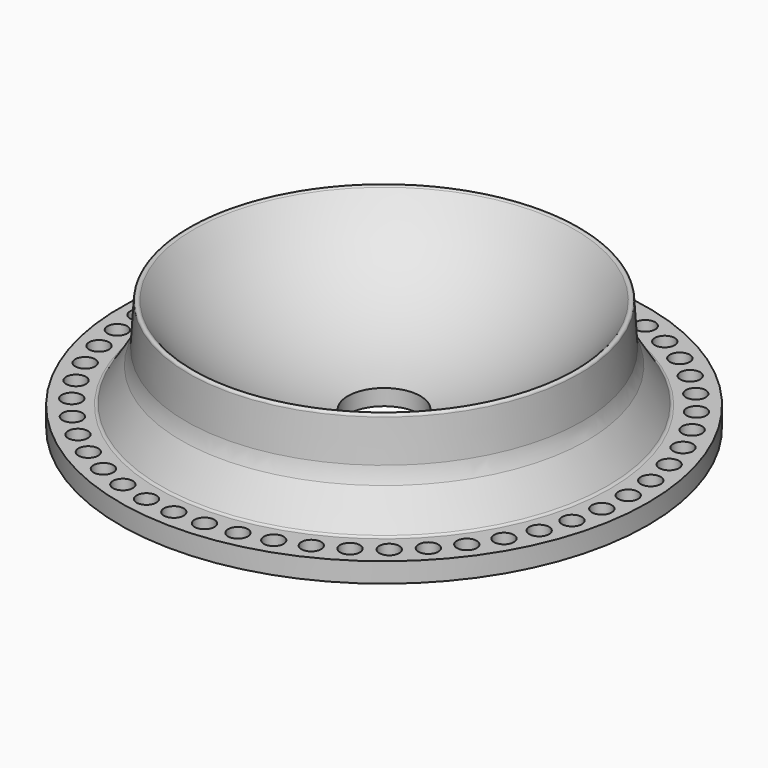
from build123d import *

# Parameters (mm, degrees)
F2_R            = 0.4
F3_R            = 5
F4_R            = 0.5
F5_R            = 5.5
F6_DEPTH        = 2.4321027845
F7_R            = 1.5
F8_DEPTH        = 3
F8_COPIES_COUNT = 50


# Not quite as in the source:
# - a pattern or mirror of a feature is missing from the dataset's text; its kind, count and spacing are read off the source's solid


with BuildPart() as f1:
    # F0 (on Front) → F1 (revolve)
    with BuildSketch(Plane.XZ):
        with BuildLine():
            Line((0, 2), (0, 0))
            Line((0, 0), (40, 0))
            Line((40, 0), (40, 3))
            Line((40, 3), (34, 3))
            Line((34, 3), (30.0883166492, 9.3437703326))
            Line((30.0883166492, 9.3437703326), (29.5567251231, 18))
            ThreePointArc((29.5567251231, 18), (16.8047612301, 6.2566432227), (0, 2))
        make_face()
    revolve(axis=Axis((0, 0, 1), (0, 0, -1)))

    # F2
    f2_edges = [f1.edges().sort_by_distance(p)[0] for p in [
        (-29.556725, 0, 18),
    ]]
    fillet(f2_edges, radius=F2_R)

    # F3
    f3_edges = [f1.edges().sort_by_distance(p)[0] for p in [
        (-30.088317, 0, 9.34377),
    ]]
    fillet(f3_edges, radius=F3_R)

    # F4
    f4_edges = [f1.edges().sort_by_distance(p)[0] for p in [
        (-34, 0, 3),
    ]]
    fillet(f4_edges, radius=F4_R)

    # F5 (on face) → F6 (cut, through all)
    with BuildSketch(Plane(origin=(0, 0, 0), x_dir=(1, 0, 0), z_dir=(0, 0, -1))):
        Circle(F5_R)
    extrude(amount=-F6_DEPTH, mode=Mode.SUBTRACT)

    # F7 (on face) → F8 (cut, through all)
    with BuildSketch(Plane.XY.offset(3)):
        with Locations((37, 0)):
            Circle(F7_R)
    f8 = extrude(amount=-F8_DEPTH, mode=Mode.SUBTRACT)

    # F8_copies: F8 ×50 about axis
    f8_copies_axis = Axis((0, 0, 0), (0, 0, 1))
    for i in range(1, F8_COPIES_COUNT):
        add(f8.rotate(f8_copies_axis, i * 360 / F8_COPIES_COUNT), mode=Mode.SUBTRACT)


solid = f1.part
